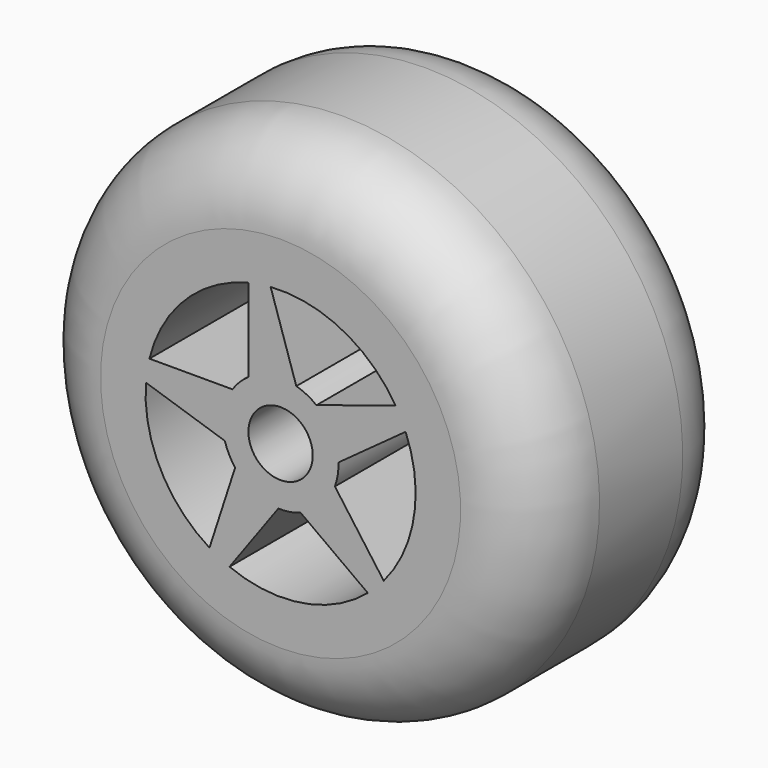
from build123d import *

# Parameters (mm, degrees)
F3_R     = 1.5875
F4_DEPTH = 12.7
F6_DEPTH = 25.4


# Not quite as in the source:
# - a fillet or chamfer that OpenCascade refuses, or shapes differently, is made with other operations: its cross-section is extruded or revolved along the edge and cut away or added


with BuildPart() as f1:
    # F0 (on Right) → F1 (revolve)
    with BuildSketch(Plane.YZ):
        Polygon((0, 12.7), (0, 0), (11.1125, 0), (11.1125, 7.9375), (12.7, 9.525), (12.7, 12.7), align=None)
    revolve(axis=Axis((0, 5.55625, 0), (0, -1, 0)))

    # F2: fillet of radius 3.81 on 2 edges, made by hand

    # F2_s1 → F2_t2 (revolve, cut)
    with BuildSketch(Plane.YZ):
        with BuildLine():
            ThreePointArc((0, 8.89), (1.1159231637, 11.5840768363), (3.81, 12.7))
            Line((3.81, 12.7), (0, 12.7))
            Line((0, 12.7), (0, 8.89))
        make_face()
    revolve(axis=Axis((0, 0, 0), (0, -1, 0)), mode=Mode.SUBTRACT)

    # F2_s3 → F2_t4 (revolve, cut)
    with BuildSketch(Plane.YZ):
        with BuildLine():
            ThreePointArc((12.7, 9.525), (11.4026337626, 11.7999355663), (8.9432893377, 12.7))
            Line((8.9432893377, 12.7), (12.7, 12.7))
            Line((12.7, 12.7), (12.7, 9.525))
        make_face()
    revolve(axis=Axis((0, 12.7, 0), (0, -1, 0)), mode=Mode.SUBTRACT)

    # F3 (on face) → F4 (cut)
    with BuildSketch(Plane(origin=(0, 11.1125, 0), x_dir=(-1, 0, 0), z_dir=(0, 1, 0))):
        Circle(F3_R)
    extrude(amount=-F4_DEPTH, mode=Mode.SUBTRACT)

    # F5 (on face) → F6 (cut)
    with BuildSketch(Plane(origin=(0, 11.1125, 0), x_dir=(-1, 0, 0), z_dir=(0, 1, 0))):
        with BuildLine():
            Line((-5.668244305, 3.5109204987), (-1.7691005725, 2.2440119016))
            ThreePointArc((-1.7691005725, 2.2440119016), (-1.297277853, 2.5460511429), (-0.7755925376, 2.7502295296))
            Line((-0.7755925376, 2.7502295296), (0.4913160595, 6.6493732622))
            ThreePointArc((0.4913160595, 6.6493732622), (-3.026981657, 5.940786), (-5.668244305, 3.5109204987))
        make_face()
        with BuildLine():
            ThreePointArc((1.5875, 2.3759524406), (2.0205576272, 2.0205576272), (2.3759524406, 1.5875))
            Line((2.3759524406, 1.5875), (6.4757547823, 1.5875))
            ThreePointArc((6.4757547823, 1.5875), (4.7146344636, 4.7146344636), (1.5875, 6.4757547823))
            Line((1.5875, 6.4757547823), (1.5875, 2.3759524406))
        make_face()
        with BuildLine():
            Line((-5.090667637, -4.3058865822), (-2.6808642833, -0.9890768143))
            ThreePointArc((-2.6808642833, -0.9890768143), (-2.8223194333, -0.4470114839), (-2.8552949903, 0.1122353262))
            Line((-2.8552949903, 0.1122353262), (-6.1721047583, 2.5220386799))
            ThreePointArc((-6.1721047583, 2.5220386799), (-6.5854120109, -1.0430267957), (-5.090667637, -4.3058865822))
        make_face()
        with BuildLine():
            Line((2.5220386799, -6.1721047583), (0.1122353262, -2.8552949903))
            ThreePointArc((0.1122353262, -2.8552949903), (-0.4470114839, -2.8223194333), (-0.9890768143, -2.6808642833))
            Line((-0.9890768143, -2.6808642833), (-4.3058865822, -5.090667637))
            ThreePointArc((-4.3058865822, -5.090667637), (-1.0430267957, -6.5854120109), (2.5220386799, -6.1721047583))
        make_face()
        with BuildLine():
            Line((6.6493732622, 0.4913160595), (2.7502295296, -0.7755925376))
            ThreePointArc((2.7502295296, -0.7755925376), (2.5460511429, -1.297277853), (2.2440119016, -1.7691005725))
            Line((2.2440119016, -1.7691005725), (3.5109204987, -5.668244305))
            ThreePointArc((3.5109204987, -5.668244305), (5.940786, -3.026981657), (6.6493732622, 0.4913160595))
        make_face()
    extrude(amount=-F6_DEPTH, mode=Mode.SUBTRACT)


solid = f1.part
